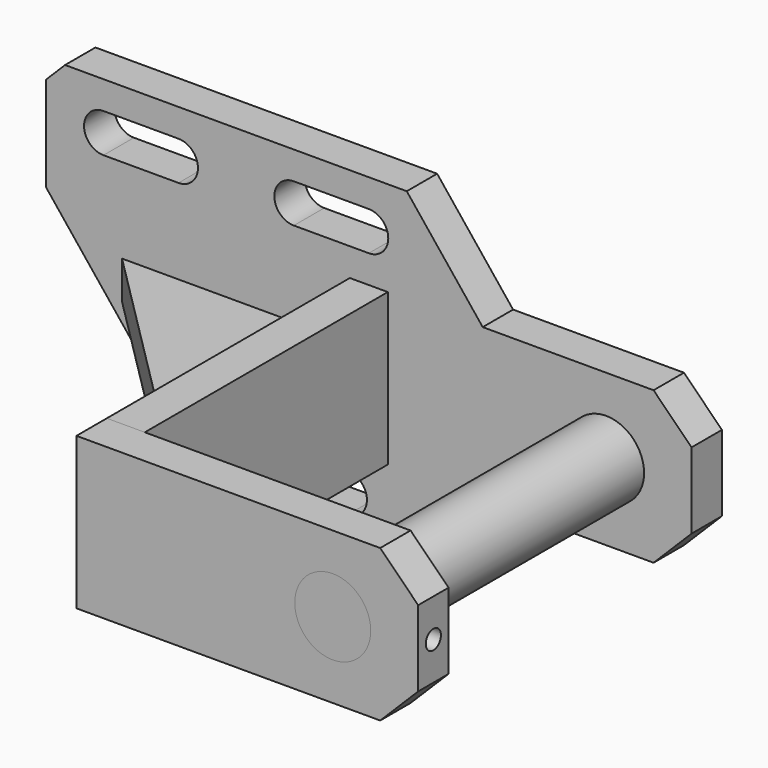
from build123d import *

# Parameters (mm, degrees)
F1_DEPTH   = 25.4
F2_R       = 25.4
F3_DEPTH   = 25.4
F4_W       = 25.4
F4_H       = 101.6
F5_DEPTH   = 203.2
F6_W       = 228.6
F6_H       = 101.6
F7_DEPTH   = 25.4
F8_R       = 25.4
F9_DEPTH   = 25.4
F12_DEPTH  = 12.7
F13_SIZE   = 12.7
F14_SIZE   = 25.4
F14_2_SIZE = 25.4
F15_SIZE   = 12.7
F16_DEPTH  = 254
F17_R      = 6.35
F18_DEPTH  = 32.5575558516
F20_DEPTH  = 25.4


with BuildPart() as f1:
    # F0 (on Front) → F1 (new body)
    with BuildSketch(Plane.XZ):
        Polygon((25.4, 107.95), (-215.9, 107.95), (-215.9, 31.75), (-104.14, -107.95), (25.4, -107.95), (76.2, -57.15), (215.9, -57.15), (215.9, 44.45), (76.2, 44.45), align=None)
    extrude(amount=F1_DEPTH)

    # F2 (on face) → F3 (cut)
    with BuildSketch(Plane.XZ.offset(25.4)):
        with Locations((158.75, -6.35)):
            Circle(F2_R)
    extrude(amount=-F3_DEPTH, mode=Mode.SUBTRACT)

    # F14
    f14_edges = [f1.edges().sort_by_distance(p)[0] for p in [
        (215.9, -12.7, -57.15),
        (215.9, -12.7, 44.45),
    ]]
    chamfer(f14_edges, length=F14_SIZE)

    # F15
    f15_edges = [f1.edges().sort_by_distance(p)[0] for p in [
        (-215.9, -12.7, 107.95),
    ]]
    chamfer(f15_edges, length=F15_SIZE)

    # F19 (on face) → F20 (cut)
    with BuildSketch(Plane.XZ.offset(25.4)):
        with BuildLine():
            Line((-127.3175, 89.2175), (-177.4825, 89.2175))
            ThreePointArc((-177.4825, 89.2175), (-190.5, 76.2), (-177.4825, 63.1825))
            Line((-177.4825, 63.1825), (-127.3175, 63.1825))
            ThreePointArc((-127.3175, 63.1825), (-114.3, 76.2), (-127.3175, 89.2175))
        make_face()
        with BuildLine():
            Line((0, 89.2175), (-50.165, 89.2175))
            ThreePointArc((-50.165, 89.2175), (-63.1825, 76.2), (-50.165, 63.1825))
            Line((-50.165, 63.1825), (0, 63.1825))
            ThreePointArc((0, 63.1825), (13.0175, 76.2), (0, 89.2175))
        make_face()
        with BuildLine():
            Line((-14.2875, -69.5325), (-64.4525, -69.5325))
            ThreePointArc((-64.4525, -69.5325), (-77.47, -82.55), (-64.4525, -95.5675))
            Line((-64.4525, -95.5675), (-14.2875, -95.5675))
            ThreePointArc((-14.2875, -95.5675), (-1.27, -82.55), (-14.2875, -69.5325))
        make_face()
    extrude(amount=-F20_DEPTH, mode=Mode.SUBTRACT)


with BuildPart() as f5:
    # F4 (on face) → F5 (new body)
    with BuildSketch(Plane.XZ.offset(25.4)):
        with Locations((0, -6.35)):
            Rectangle(F4_W, F4_H)
    extrude(amount=F5_DEPTH)


with BuildPart() as f7:
    # F6 (on face) → F7 (new body)
    with BuildSketch(Plane.XZ.offset(228.6)):
        with Locations((101.6, -6.35)):
            Rectangle(F6_W, F6_H)
    extrude(amount=F7_DEPTH)

    # F8 (on face) → F9 (cut)
    with BuildSketch(Plane.XZ.offset(254)):
        with Locations((158.75, -6.35)):
            Circle(F8_R)
    extrude(amount=-F9_DEPTH, mode=Mode.SUBTRACT)

    # F14#2
    f14_2_edges = [f7.edges().sort_by_distance(p)[0] for p in [
        (215.9, -241.3, 44.45),
        (215.9, -241.3, -57.15),
    ]]
    chamfer(f14_2_edges, length=F14_2_SIZE)

    # F17 (on face) → F18 (cut, through all)
    with BuildSketch(Plane.YZ.offset(215.9)):
        with Locations((-241.3, -6.35)):
            Circle(F17_R)
    extrude(amount=-F18_DEPTH, mode=Mode.SUBTRACT)


with BuildPart() as f12:
    # F11 (on mid) → F12 (new body, symmetric)
    with BuildSketch(Plane.XY.offset(-6.35)):
        Polygon((-12.7, -25.4), (-165.1, -25.4), (-12.7, -177.8), align=None)
    extrude(amount=F12_DEPTH, both=True)

    # F13
    f13_edges = [f12.edges().sort_by_distance(p)[0] for p in [
        (-12.7, -25.4, -6.35),
    ]]
    chamfer(f13_edges, length=F13_SIZE)


with BuildPart() as f16:
    # F8 (on face) → F16 (new body, through all)
    with BuildSketch(Plane.XZ.offset(254)):
        with Locations((158.75, -6.35)):
            Circle(F8_R)
    extrude(amount=-F16_DEPTH)


solid = Compound([f1.part, f5.part, f7.part, f12.part, f16.part])
